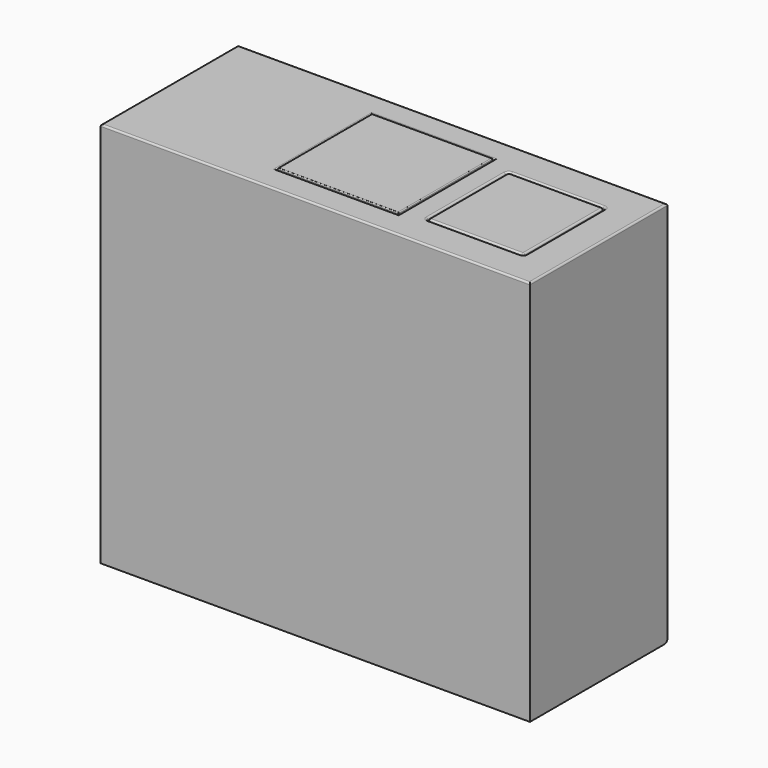
from build123d import *

# Parameters (mm, degrees)
F1_W        = 500
F1_H        = 200
F2_DEPTH    = 450
F3_W        = 114.8297786713
F3_H        = 120.7839138806
F4_DEPTH    = 10
F5_T1_DEPTH = 19.9997500031
F5_T3_DEPTH = 519.9995000063
F7_DEPTH    = 10
F8_R        = 2
F9_W        = 142.3365101218
F9_H        = 139.1178444028
F10_DEPTH   = 5
F11_W       = 140.5770033598
F11_H       = 137.1815949678
F12_DEPTH   = 6
F13_R       = 1
F14_R       = 2
F15_W       = 71.6344714165
F15_H       = 192.6967278123
F16_DEPTH   = 127
F17_W       = 191.3057491183
F17_H       = 2.1015560806
F17_H_2     = 20.5821128011
F18_DEPTH   = 76.5471703


# Not quite as in the source:
# - a fillet or chamfer that OpenCascade refuses, or shapes differently, is made with other operations: its cross-section is extruded or revolved along the edge and cut away or added
# - an extrude ends at something that could not be found from the text; its depth is read off the source's solid


with BuildPart() as f2:
    # F1 (on offset) → F2 (new body)
    with BuildSketch(Plane.XY.offset(50.8)):
        with Locations((16.9582420111, -6.3602398952)):
            Rectangle(F1_W, F1_H)
    extrude(amount=F2_DEPTH)

    # F3 (on face) → F4 (cut)
    with BuildSketch(Plane.XY.offset(500.8)):
        with Locations((171.4461296797, -7.3848497123)):
            Rectangle(F3_W, F3_H)
    extrude(amount=-F4_DEPTH, mode=Mode.SUBTRACT)

    # F5: fillet of radius 4 on 5 edges, made by hand

    # F5_s2 → F5_t1 (join)
    with BuildSketch(Plane.XY.offset(480.8002499969)):
        with BuildLine():
            ThreePointArc((228.8611190153, 49.007207228), (227.6895461401, 51.8356343528), (224.8611190153, 53.007207228))
            Line((224.8611190153, 53.007207228), (224.8611190153, 53.087207228))
            ThreePointArc((224.8611190153, 53.087207228), (226.8610690153, 53.087107228), (228.8610190153, 53.087107228))
            Line((228.8610190153, 53.087107228), (228.9410190153, 53.007107228))
            ThreePointArc((228.9410190153, 53.007107228), (228.9410190153, 51.007157228), (228.9411190153, 49.007207228))
            Line((228.9411190153, 49.007207228), (228.8611190153, 49.007207228))
        make_face()
        with BuildLine():
            ThreePointArc((228.8611190153, -63.7769066525), (227.6895461401, -66.6053337773), (224.8611190153, -67.7769066525))
            Line((224.8611190153, -67.7769066525), (224.8611190153, -67.8569066525))
            ThreePointArc((224.8611190153, -67.8569066525), (226.8610690153, -67.8568066525), (228.8610190153, -67.8568066525))
            Line((228.8610190153, -67.8568066525), (228.9410190153, -67.7768066525))
            ThreePointArc((228.9410190153, -67.7768066525), (228.9410190153, -65.7768566525), (228.9411190153, -63.7769066525))
            Line((228.9411190153, -63.7769066525), (228.8611190153, -63.7769066525))
        make_face()
        with BuildLine():
            ThreePointArc((118.031140344, 53.007207228), (115.2027132193, 51.8356343528), (114.031140344, 49.007207228))
            Line((114.031140344, 49.007207228), (113.951140344, 49.007207228))
            ThreePointArc((113.951140344, 49.007207228), (113.951240344, 51.007157228), (113.951240344, 53.007107228))
            Line((113.951240344, 53.007107228), (114.031240344, 53.087107228))
            ThreePointArc((114.031240344, 53.087107228), (116.031190344, 53.087107228), (118.031140344, 53.087207228))
            Line((118.031140344, 53.087207228), (118.031140344, 53.007207228))
        make_face()
        with BuildLine():
            ThreePointArc((114.031140344, -63.7769066525), (115.2027132193, -66.6053337773), (118.031140344, -67.7769066525))
            Line((118.031140344, -67.7769066525), (118.031140344, -67.8569066525))
            ThreePointArc((118.031140344, -67.8569066525), (116.031190344, -67.8568066525), (114.031240344, -67.8568066525))
            Line((114.031240344, -67.8568066525), (113.951240344, -67.7768066525))
            ThreePointArc((113.951240344, -67.7768066525), (113.951240344, -65.7768566525), (113.951140344, -63.7769066525))
            Line((113.951140344, -63.7769066525), (114.031140344, -63.7769066525))
        make_face()
    extrude(amount=F5_T1_DEPTH)

    # F5_s4 → F5_t3 (cut)
    with BuildSketch(Plane.YZ.offset(-243.0415079921)):
        with BuildLine():
            ThreePointArc((93.6398601048, 54.7999), (92.4682872295, 51.9714728753), (89.6398601048, 50.7999))
            Line((89.6398601048, 50.7999), (89.6398601048, 50.7199))
            ThreePointArc((89.6398601048, 50.7199), (91.6398101048, 50.72), (93.6397601048, 50.72))
            Line((93.6397601048, 50.72), (93.7197601048, 50.8))
            ThreePointArc((93.7197601048, 50.8), (93.7197601048, 52.79995), (93.7198601048, 54.7999))
            Line((93.7198601048, 54.7999), (93.6398601048, 54.7999))
        make_face()
    extrude(amount=F5_T3_DEPTH, mode=Mode.SUBTRACT)

    # F9 (on face) → F10 (cut)
    with BuildSketch(Plane.XY.offset(500.8)):
        with Locations((18.0311240256, -5.8237947524)):
            Rectangle(F9_W, F9_H)
    extrude(amount=-F10_DEPTH, mode=Mode.SUBTRACT)

    # F14
    f14_edges = [f2.edges().sort_by_distance(p)[0] for p in [
        (266.958242, -6.36024, 500.8),
        (16.958242, -106.36024, 500.8),
        (16.958242, 93.63976, 500.8),
        (-233.041758, -6.36024, 500.8),
        (228.861019, -7.38485, 500.8),
        (227.689546, -66.605334, 500.8),
        (227.689546, 51.835634, 500.8),
        (171.44613, -67.776807, 500.8),
        (171.44613, 53.007107, 500.8),
        (115.202713, -66.605334, 500.8),
        (115.202713, 51.835634, 500.8),
        (114.03124, -7.38485, 500.8),
        (89.199379, -5.823795, 500.8),
        (18.031124, 63.735127, 500.8),
        (-53.137131, -5.823795, 500.8),
        (18.031124, -75.382717, 500.8),
    ]]
    fillet(f14_edges, radius=F14_R)

    # F15 (on face) → F16 (cut)
    with BuildSketch(Plane.XY.offset(50.8)):
        with Locations((-192.3118233681, -6.6746808589)):
            Rectangle(F15_W, F15_H)
    extrude(amount=F16_DEPTH, mode=Mode.SUBTRACT)

    # F17 (on face) → F18 (cut, through all)
    with BuildSketch(Plane(origin=(-233.0417579889, 0, 0), x_dir=(0, -1, 0), z_dir=(-1, 0, 0))):
        with Locations((6.6700465977, 49.7492219597)):
            Rectangle(F17_W, F17_H)
        with Locations((6.6700465977, 61.0910564005)):
            Rectangle(F17_W, F17_H_2)
    extrude(amount=-F18_DEPTH, mode=Mode.SUBTRACT)


with BuildPart() as f7:
    # F6 (on face) → F7 (new body)
    with BuildSketch(Plane.XY.offset(490.8)):
        with BuildLine():
            Line((224.6392856836, 51.2222974241), (117.8006191254, 51.2222974241))
            ThreePointArc((117.8006191254, 51.2222974241), (116.386405563, 50.6365109865), (115.8006191254, 49.2222974241))
            Line((115.8006191254, 49.2222974241), (115.8006191254, -63.5862987041))
            ThreePointArc((115.8006191254, -63.5862987041), (116.386405563, -65.0005122665), (117.8006191254, -65.5862987041))
            Line((117.8006191254, -65.5862987041), (224.6392856836, -65.5862987041))
            ThreePointArc((224.6392856836, -65.5862987041), (226.053499246, -65.0005122665), (226.6392856836, -63.5862987041))
            Line((226.6392856836, -63.5862987041), (226.6392856836, 49.2222974241))
            ThreePointArc((226.6392856836, 49.2222974241), (226.053499246, 50.6365109865), (224.6392856836, 51.2222974241))
        make_face()
    extrude(amount=F7_DEPTH)

    # F8
    f8_edges = [f7.edges().sort_by_distance(p)[0] for p in [
        (171.219952, 51.222297, 500.8),
        (116.386406, 50.636511, 500.8),
        (115.800619, -7.182001, 500.8),
        (116.386406, -65.000512, 500.8),
        (171.219952, -65.586299, 500.8),
        (226.053499, -65.000512, 500.8),
        (226.639286, -7.182001, 500.8),
        (226.053499, 50.636511, 500.8),
    ]]
    fillet(f8_edges, radius=F8_R)


with BuildPart() as f12:
    # F11 (on face) → F12 (new body)
    with BuildSketch(Plane.XY.offset(495.8)):
        with Locations((17.9034695029, -5.767442286)):
            Rectangle(F11_W, F11_H)
    extrude(amount=F12_DEPTH)

    # F13
    f13_edges = [f12.edges().sort_by_distance(p)[0] for p in [
        (17.90347, 62.823355, 501.8),
        (-52.385032, -5.767442, 501.8),
        (17.90347, -74.35824, 501.8),
        (88.191971, -5.767442, 501.8),
    ]]
    fillet(f13_edges, radius=F13_R)


solid = Compound([f2.part, f7.part, f12.part])
